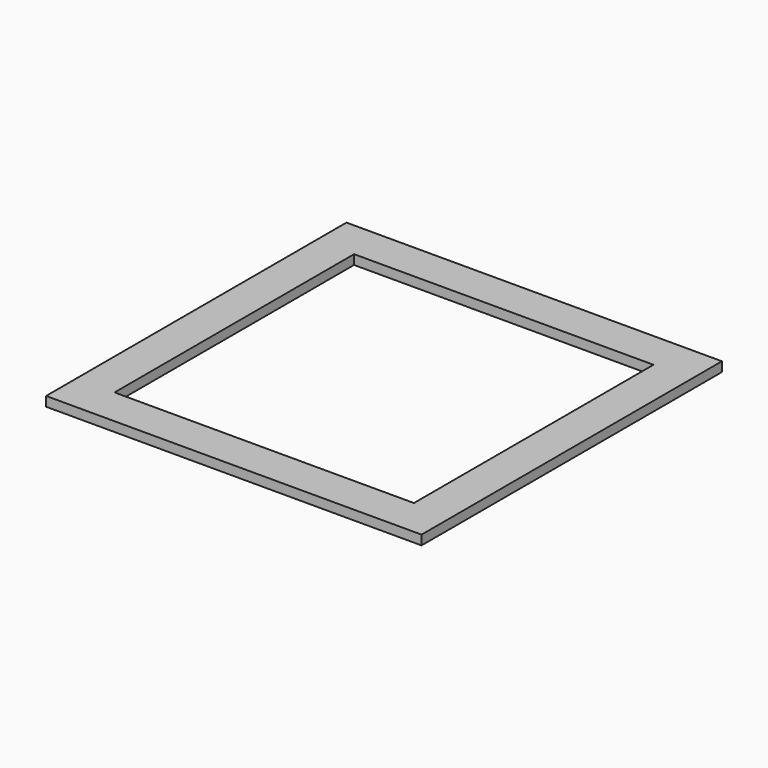
from build123d import *

# Parameters (mm, degrees)
F0_W     = 501.6
F0_H     = 501.6
F0_W_2   = 400
F0_H_2   = 400
F1_DEPTH = 12.7


# Not quite as in the source:
# - a length typed as a fraction of an inch, garbled in the dataset ("3 / 203.2 mm" for 3/8 in), is restored


with BuildPart() as f1:
    # F0 (on Top) → F1 (new body)
    with BuildSketch(Plane.XY):
        Rectangle(F0_W, F0_H)
        Rectangle(F0_W_2, F0_H_2, mode=Mode.SUBTRACT)
    extrude(amount=F1_DEPTH)


solid = f1.part
